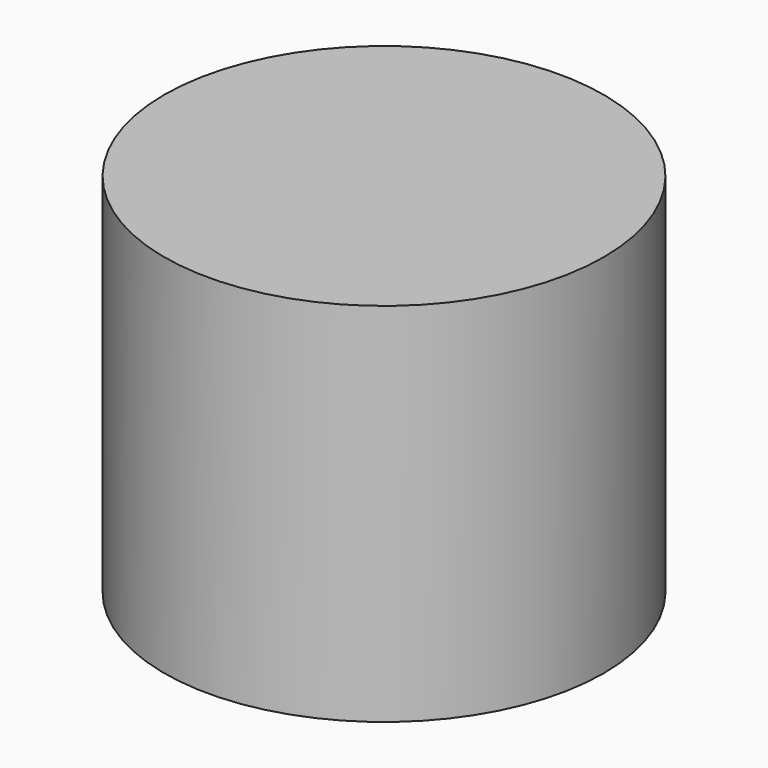
from build123d import *

# Parameters (mm, degrees)
F1_W          = 15
F1_H          = 25
F3_T          = -3
F4_DEPTH      = 12.0000001006
F4_DEPTH_BACK = 12.0000001006
F5_R          = 2.5
F6_DEPTH      = 5
F7_W          = 10
F7_H          = 7
F8_DEPTH      = 12
F8_DEPTH_BACK = 12


with BuildPart() as f2:
    # F1 (on Front) → F2 (revolve)
    with BuildSketch(Plane.XZ):
        with Locations((7.5, 64.7015325446)):
            Rectangle(F1_W, F1_H)
    revolve(axis=Axis((0, 0, 62.2015325446), (0, 0, 1)))

    # F3
    f3_openings = [f2.faces().sort_by_distance(p)[0] for p in [
        (0, 0, 52.201533),
    ]]
    offset(amount=F3_T, openings=f3_openings)

    # F0 (on Front) → F4 (join, two sides)
    with BuildSketch(Plane.XZ) as f4_sk:
        with BuildLine():
            ThreePointArc((-5, 62.2015325446), (-4.0541927813, 59.2751831307), (-1.5745916432, 57.4559386769))
            ThreePointArc((-1.5745916432, 57.4559386769), (2.9263494138, 58.1473397632), (5, 62.2015325446))
            Line((5, 62.2015325446), (5, 70.2015325446))
            Line((5, 70.2015325446), (-5, 70.2015325446))
            Line((-5, 70.2015325446), (-5, 62.2015325446))
        make_face()
        with BuildLine():
            ThreePointArc((2.5, 62.2015325446), (1.4631747069, 60.1744361539), (-0.7872958216, 59.8287356107))
            ThreePointArc((-0.7872958216, 59.8287356107), (-1.4631747069, 64.2286289352), (2.5, 62.2015325446))
        make_face(mode=Mode.SUBTRACT)
    extrude(amount=-F4_DEPTH)
    extrude(f4_sk.sketch, amount=F4_DEPTH_BACK)

    # F5 (on Front) → F6 (cut, symmetric)
    with BuildSketch(Plane.XZ):
        with BuildLine():
            Line((5, 70.2015325446), (-5, 70.2015325446))
            Line((-5, 70.2015325446), (-5, 62.2015325446))
            ThreePointArc((-5, 62.2015325446), (0, 57.2015325446), (5, 62.2015325446))
            Line((5, 62.2015325446), (5, 70.2015325446))
        make_face()
        with Locations((0, 62.2015325446)):
            Circle(F5_R, mode=Mode.SUBTRACT)
    extrude(amount=F6_DEPTH, both=True, mode=Mode.SUBTRACT)

    # F7 (on Front) → F8 (join, two sides)
    with BuildSketch(Plane.XZ) as f8_sk:
        with Locations((0, 73.7015325446)):
            Rectangle(F7_W, F7_H)
    extrude(amount=F8_DEPTH)
    extrude(f8_sk.sketch, amount=-F8_DEPTH_BACK)


solid = f2.part
